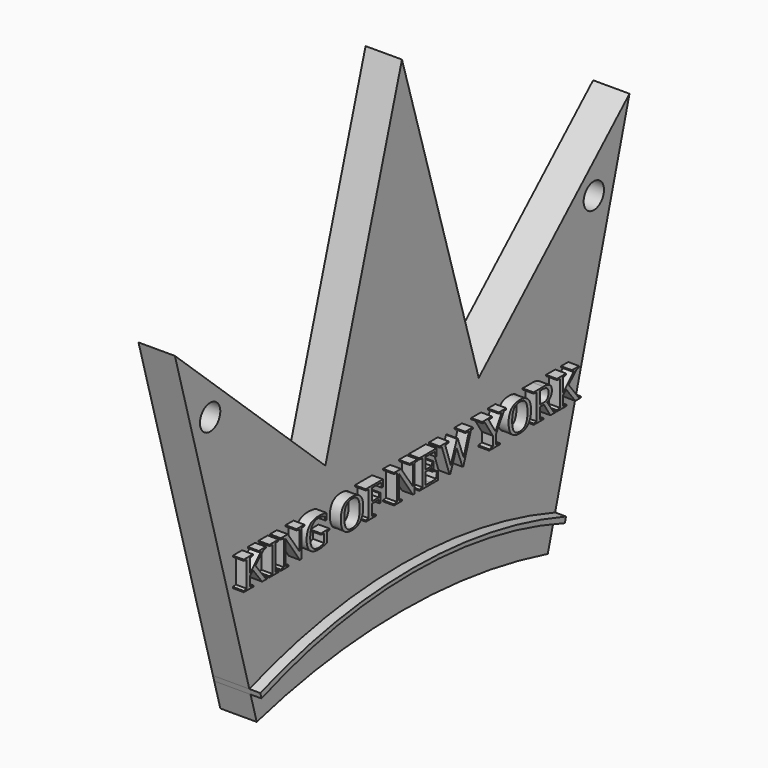
from build123d import *

# Parameters (mm, degrees)
F0_R         = 0.889
F1_DEPTH     = 2.54
F0_TEXT_SIZE = 3.0652309457
F2_DEPTH     = 3.302


# Not quite as in the source:
# - a feature names something its author has since deleted; it is built from what else it names
# - Text() gives the source's letters only with a copy of the font that has no kerning and outlines rounded to 1/6400 em; it was checked with that copy


with BuildPart() as f1:
    # F0 (on Right) → F1 (new body)
    with BuildSketch(Plane.YZ):
        with BuildLine():
            Line((-58.5731928543, 116.2585045769), (-59.2243112864, 116.8579392082))
            Line((-59.2243112864, 116.8579392082), (-52.7272009337, 93.7439392082))
            ThreePointArc((-52.7272009337, 93.7439392082), (-39.3847965103, 96.0063092306), (-26.0423920869, 93.7439392082))
            Line((-26.0423920869, 93.7439392082), (-19.5532767107, 116.8414972067))
            Line((-19.5532767107, 116.8414972067), (-32.7116451349, 104.7276000479))
            Line((-32.7116451349, 104.7276000479), (-39.408698678, 127.0142197609))
            Line((-39.408698678, 127.0142197609), (-46.0932555591, 104.7691867476))
            Line((-46.0932555591, 104.7691867476), (-58.5731928543, 116.2585045769))
        make_face()
        Polygon((-52.8586438159, 102.5280816539), (-52.230271472, 102.5280816539), (-52.230271472, 102.4485772262), (-52.4620795622, 102.4097828971), (-53.147446044, 101.7392636277), (-52.2901392639, 100.6405699106), (-52.073178386, 100.6003387544), (-52.073178386, 100.5208343267), (-52.5640942797, 100.5208343267), (-53.3495597095, 101.5357131352), (-53.6206410713, 101.3187522573), (-53.6206410713, 100.6405699106), (-53.3332756701, 100.6003387544), (-53.3332756701, 100.5208343267), (-54.1671142758, 100.5208343267), (-54.1671142758, 100.6003387544), (-53.9094432994, 100.6405699106), (-53.9094432994, 102.4097828971), (-54.1671142758, 102.4485772262), (-54.1671142758, 102.5280816539), (-53.3629700949, 102.5280816539), (-53.3629700949, 102.4485772262), (-53.6206410713, 102.4097828971), (-53.6206410713, 101.4638717849), (-52.6598827467, 102.4097828971), (-52.8586438159, 102.4485772262), align=None, mode=Mode.SUBTRACT)
        Polygon((-51.3858961349, 102.4097828971), (-51.3858961349, 100.6405699106), (-51.1287041008, 100.6003387544), (-51.1287041008, 100.5208343267), (-51.9309325124, 100.5208343267), (-51.9309325124, 100.6003387544), (-51.6732615361, 100.6405699106), (-51.6732615361, 102.4097828971), (-51.9309325124, 102.4485772262), (-51.9309325124, 102.5280816539), (-51.1287041008, 102.5280816539), (-51.1287041008, 102.4485772262), align=None, mode=Mode.SUBTRACT)
        Polygon((-49.2924391874, 101.0419235875), (-49.2924391874, 102.4097828971), (-49.5616047798, 102.4485772262), (-49.5616047798, 102.5280816539), (-48.8776751251, 102.5280816539), (-48.8776751251, 102.4485772262), (-49.1348671591, 102.4097828971), (-49.1348671591, 100.5208343267), (-49.280465629, 100.5208343267), (-50.5180526234, 102.3259679884), (-50.5180526234, 100.6405699106), (-50.2484080886, 100.6003387544), (-50.2484080886, 100.5208343267), (-50.9328166857, 100.5208343267), (-50.9328166857, 100.6003387544), (-50.6751457093, 100.6405699106), (-50.6751457093, 102.4097828971), (-50.9328166857, 102.4485772262), (-50.9328166857, 102.5280816539), (-50.3250388623, 102.5280816539), align=None, mode=Mode.SUBTRACT)
        with BuildLine():
            Line((-46.8852750103, 101.2780421588), (-46.8852750103, 100.6257226982))
            add(Edge.make_bspline(
                [(-46.8852750103, 100.6257226982), (-47.059131078, 100.5687285603), (-47.24615806, 100.5296947599)],
                knots=[0, 0, 0, 1, 1, 1], degree=2))
            add(Edge.make_bspline(
                [(-47.24615806, 100.5296947599), (-47.4331850419, 100.4906609596), (-47.6487090928, 100.4906609596)],
                knots=[0, 0, 0, 1, 1, 1], degree=2))
            add(Edge.make_bspline(
                [(-47.6487090928, 100.4906609596), (-48.1367513324, 100.4906609596), (-48.40903005, 100.7543187152)],
                knots=[0, 0, 0, 1, 1, 1], degree=2))
            add(Edge.make_bspline(
                [(-48.40903005, 100.7543187152), (-48.6813087676, 101.0179764708), (-48.6813087676, 101.501229287)],
                knots=[0, 0, 0, 1, 1, 1], degree=2))
            add(Edge.make_bspline(
                [(-48.6813087676, 101.501229287), (-48.6813087676, 102.0280658558), (-48.4171720697, 102.2893288997)],
                knots=[0, 0, 0, 1, 1, 1], degree=2))
            add(Edge.make_bspline(
                [(-48.4171720697, 102.2893288997), (-48.1530353718, 102.5505919436), (-47.6429617847, 102.5505919436)],
                knots=[0, 0, 0, 1, 1, 1], degree=2))
            add(Edge.make_bspline(
                [(-47.6429617847, 102.5505919436), (-47.2775287829, 102.5505919436), (-46.9379586672, 102.4605507846)],
                knots=[0, 0, 0, 1, 1, 1], degree=2))
            Line((-46.9379586672, 102.4605507846), (-46.9379586672, 102.0295026829))
            Line((-46.9379586672, 102.0295026829), (-47.0380576153, 102.0295026829))
            Line((-47.0380576153, 102.0295026829), (-47.0787677138, 102.2780737549))
            add(Edge.make_bspline(
                [(-47.0787677138, 102.2780737549), (-47.1817403159, 102.3513519322), (-47.3261414299, 102.391104146)],
                knots=[0, 0, 0, 1, 1, 1], degree=2))
            add(Edge.make_bspline(
                [(-47.3261414299, 102.391104146), (-47.470542544, 102.4308563598), (-47.6309882263, 102.4308563598)],
                knots=[0, 0, 0, 1, 1, 1], degree=2))
            add(Edge.make_bspline(
                [(-47.6309882263, 102.4308563598), (-48.0141420946, 102.4308563598), (-48.1913507586, 102.2024008659)],
                knots=[0, 0, 0, 1, 1, 1], degree=2))
            add(Edge.make_bspline(
                [(-48.1913507586, 102.2024008659), (-48.3685594227, 101.973945372), (-48.3685594227, 101.5041029411)],
                knots=[0, 0, 0, 1, 1, 1], degree=2))
            add(Edge.make_bspline(
                [(-48.3685594227, 101.5041029411), (-48.3685594227, 101.0625181079), (-48.1860823929, 100.8343020852)],
                knots=[0, 0, 0, 1, 1, 1], degree=2))
            add(Edge.make_bspline(
                [(-48.1860823929, 100.8343020852), (-48.0036053632, 100.6060860624), (-47.6458354387, 100.6060860624)],
                knots=[0, 0, 0, 1, 1, 1], degree=2))
            add(Edge.make_bspline(
                [(-47.6458354387, 100.6060860624), (-47.5198736046, 100.6060860624), (-47.3821776832, 100.6360199584)],
                knots=[0, 0, 0, 1, 1, 1], degree=2))
            add(Edge.make_bspline(
                [(-47.3821776832, 100.6360199584), (-47.2444817618, 100.6659538543), (-47.1726404115, 100.7081007798)],
                knots=[0, 0, 0, 1, 1, 1], degree=2))
            Line((-47.1726404115, 100.7081007798), (-47.1726404115, 101.2780421588))
            Line((-47.1726404115, 101.2780421588), (-47.4303113879, 101.3173154303))
            Line((-47.4303113879, 101.3173154303), (-47.4303113879, 101.3977777426))
            Line((-47.4303113879, 101.3977777426), (-46.6893875952, 101.3977777426))
            Line((-46.6893875952, 101.3977777426), (-46.6893875952, 101.3173154303))
            Line((-46.6893875952, 101.3173154303), (-46.8852750103, 101.2780421588))
        make_face(mode=Mode.SUBTRACT)
        with BuildLine():
            add(Edge.make_bspline(
                [(-45.4498848315, 100.7519240035), (-45.7013295575, 101.0131870474), (-45.7013295575, 101.5266132308)],
                knots=[0, 0, 0, 1, 1, 1], degree=2))
            add(Edge.make_bspline(
                [(-45.7013295575, 101.5266132308), (-45.7013295575, 102.5505919436), (-44.7214135396, 102.5505919436)],
                knots=[0, 0, 0, 1, 1, 1], degree=2))
            add(Edge.make_bspline(
                [(-44.7214135396, 102.5505919436), (-44.2362449539, 102.5505919436), (-43.9879133531, 102.2907657267)],
                knots=[0, 0, 0, 1, 1, 1], degree=2))
            add(Edge.make_bspline(
                [(-43.9879133531, 102.2907657267), (-43.7395817523, 102.0309395099), (-43.7395817523, 101.5266132308)],
                knots=[0, 0, 0, 1, 1, 1], degree=2))
            add(Edge.make_bspline(
                [(-43.7395817523, 101.5266132308), (-43.7395817523, 101.0146238744), (-43.9910264783, 100.752642417)],
                knots=[0, 0, 0, 1, 1, 1], degree=2))
            add(Edge.make_bspline(
                [(-43.9910264783, 100.752642417), (-44.2424712043, 100.4906609596), (-44.7214135396, 100.4906609596)],
                knots=[0, 0, 0, 1, 1, 1], degree=2))
            add(Edge.make_bspline(
                [(-44.7214135396, 100.4906609596), (-45.1984401055, 100.4906609596), (-45.4498848315, 100.7519240035)],
                knots=[0, 0, 0, 1, 1, 1], degree=2))
        make_face(mode=Mode.SUBTRACT)
        with BuildLine():
            Line((-42.3880064821, 101.4217248594), (-42.9790213238, 101.4217248594))
            Line((-42.9790213238, 101.4217248594), (-42.9790213238, 100.6405699106))
            Line((-42.9790213238, 100.6405699106), (-42.6451985162, 100.6003387544))
            Line((-42.6451985162, 100.6003387544), (-42.6451985162, 100.5208343267))
            Line((-42.6451985162, 100.5208343267), (-43.5058578926, 100.5208343267))
            Line((-43.5058578926, 100.5208343267), (-43.5058578926, 100.6003387544))
            Line((-43.5058578926, 100.6003387544), (-43.267823552, 100.6405699106))
            Line((-43.267823552, 100.6405699106), (-43.267823552, 102.4097828971))
            Line((-43.267823552, 102.4097828971), (-43.5254945284, 102.4485772262))
            Line((-43.5254945284, 102.4485772262), (-43.5254945284, 102.5280816539))
            Line((-43.5254945284, 102.5280816539), (-42.0196998263, 102.5280816539))
            Line((-42.0196998263, 102.5280816539), (-42.0196998263, 102.0477024916))
            Line((-42.0196998263, 102.0477024916), (-42.1183619474, 102.0477024916))
            Line((-42.1183619474, 102.0477024916), (-42.1662561809, 102.3724253949))
            add(Edge.make_bspline(
                [(-42.1662561809, 102.3724253949), (-42.3338859982, 102.3930199153), (-42.6514247665, 102.3930199153)],
                knots=[0, 0, 0, 1, 1, 1], degree=2))
            Line((-42.6514247665, 102.3930199153), (-42.9790213238, 102.3930199153))
            Line((-42.9790213238, 102.3930199153), (-42.9790213238, 101.5567865979))
            Line((-42.9790213238, 101.5567865979), (-42.3880064821, 101.5567865979))
            Line((-42.3880064821, 101.5567865979), (-42.3415490756, 101.7962577656))
            Line((-42.3415490756, 101.7962577656), (-42.2500710896, 101.7962577656))
            Line((-42.2500710896, 101.7962577656), (-42.2500710896, 101.1793800377))
            Line((-42.2500710896, 101.1793800377), (-42.3415490756, 101.1793800377))
            Line((-42.3415490756, 101.1793800377), (-42.3880064821, 101.4217248594))
        make_face(mode=Mode.SUBTRACT)
        Polygon((-39.4142535224, 101.0419235875), (-39.4142535224, 102.4097828971), (-39.6834191148, 102.4485772262), (-39.6834191148, 102.5280816539), (-38.9994894601, 102.5280816539), (-38.9994894601, 102.4485772262), (-39.2566814941, 102.4097828971), (-39.2566814941, 100.5208343267), (-39.402279964, 100.5208343267), (-40.6398669584, 102.3259679884), (-40.6398669584, 100.6405699106), (-40.3702224236, 100.6003387544), (-40.3702224236, 100.5208343267), (-41.0546310207, 100.5208343267), (-41.0546310207, 100.6003387544), (-40.7969600443, 100.6405699106), (-40.7969600443, 102.4097828971), (-41.0546310207, 102.4485772262), (-41.0546310207, 102.5280816539), (-40.4468531973, 102.5280816539), align=None, mode=Mode.SUBTRACT)
        with BuildLine():
            Line((-38.8409595471, 100.5208343267), (-38.8409595471, 100.6003387544))
            Line((-38.8409595471, 100.6003387544), (-38.5832885707, 100.6405699106))
            Line((-38.5832885707, 100.6405699106), (-38.5832885707, 102.4097828971))
            Line((-38.5832885707, 102.4097828971), (-38.8409595471, 102.4485772262))
            Line((-38.8409595471, 102.4485772262), (-38.8409595471, 102.5280816539))
            Line((-38.8409595471, 102.5280816539), (-37.335164845, 102.5280816539))
            Line((-37.335164845, 102.5280816539), (-37.335164845, 102.0477024916))
            Line((-37.335164845, 102.0477024916), (-37.4338269661, 102.0477024916))
            Line((-37.4338269661, 102.0477024916), (-37.4817211996, 102.3724253949))
            add(Edge.make_bspline(
                [(-37.4817211996, 102.3724253949), (-37.6493510169, 102.3930199153), (-37.9668897852, 102.3930199153)],
                knots=[0, 0, 0, 1, 1, 1], degree=2))
            Line((-37.9668897852, 102.3930199153), (-38.2944863425, 102.3930199153))
            Line((-38.2944863425, 102.3930199153), (-38.2944863425, 101.6089913125))
            Line((-38.2944863425, 101.6089913125), (-37.7528025613, 101.6089913125))
            Line((-37.7528025613, 101.6089913125), (-37.7063451548, 101.8484624801))
            Line((-37.7063451548, 101.8484624801), (-37.6105566878, 101.8484624801))
            Line((-37.6105566878, 101.8484624801), (-37.6105566878, 101.2315847523))
            Line((-37.6105566878, 101.2315847523), (-37.7063451548, 101.2315847523))
            Line((-37.7063451548, 101.2315847523), (-37.7528025613, 101.4744085163))
            Line((-37.7528025613, 101.4744085163), (-38.2944863425, 101.4744085163))
            Line((-38.2944863425, 101.4744085163), (-38.2944863425, 100.655417123))
            Line((-38.2944863425, 100.655417123), (-37.8993589159, 100.655417123))
            add(Edge.make_bspline(
                [(-37.8993589159, 100.655417123), (-37.5133313937, 100.655417123), (-37.3935958099, 100.6793642397)],
                knots=[0, 0, 0, 1, 1, 1], degree=2))
            Line((-37.3935958099, 100.6793642397), (-37.3083440742, 101.0505445496))
            Line((-37.3083440742, 101.0505445496), (-37.2092030108, 101.0505445496))
            Line((-37.2092030108, 101.0505445496), (-37.2379395509, 100.5208343267))
            Line((-37.2379395509, 100.5208343267), (-38.8409595471, 100.5208343267))
        make_face(mode=Mode.SUBTRACT)
        Polygon((-34.3446489035, 102.4097828971), (-35.0003209605, 100.4743769202), (-35.0798253882, 100.4743769202), (-35.6004357066, 101.8575623845), (-36.1349353528, 100.4743769202), (-36.2144397805, 100.4743769202), (-36.8787327995, 102.4097828971), (-37.0540256942, 102.4485772262), (-37.0540256942, 102.5280816539), (-36.2877179577, 102.5280816539), (-36.2877179577, 102.4485772262), (-36.5822674939, 102.4097828971), (-36.1047619857, 100.995466181), (-35.5645150315, 102.3872726073), (-35.4974631045, 102.3872726073), (-34.9763738438, 100.995466181), (-34.5213786253, 102.4097828971), (-34.8341279702, 102.4485772262), (-34.8341279702, 102.5280816539), (-34.1698349512, 102.5280816539), (-34.1698349512, 102.4485772262), align=None, mode=Mode.SUBTRACT)
        Polygon((-31.4815316233, 102.4097828971), (-32.1429509883, 101.3110891799), (-32.1429509883, 100.6405699106), (-31.8244543353, 100.6003387544), (-31.8244543353, 100.5208343267), (-32.7507288118, 100.5208343267), (-32.7507288118, 100.6003387544), (-32.4317532165, 100.6405699106), (-32.4317532165, 101.3019892756), (-33.136756334, 102.4097828971), (-33.3628171162, 102.4485772262), (-33.3628171162, 102.5280816539), (-32.5141312981, 102.5280816539), (-32.5141312981, 102.4485772262), (-32.7837758329, 102.4097828971), (-32.2076082036, 101.4830294783), (-31.659698172, 102.4097828971), (-31.914016552, 102.4485772262), (-31.914016552, 102.5280816539), (-31.2616970914, 102.5280816539), (-31.2616970914, 102.4485772262), align=None, mode=Mode.SUBTRACT)
        with BuildLine():
            add(Edge.make_bspline(
                [(-30.8062229306, 100.7519240035), (-31.0576676566, 101.0131870474), (-31.0576676566, 101.5266132308)],
                knots=[0, 0, 0, 1, 1, 1], degree=2))
            add(Edge.make_bspline(
                [(-31.0576676566, 101.5266132308), (-31.0576676566, 102.5505919436), (-30.0777516386, 102.5505919436)],
                knots=[0, 0, 0, 1, 1, 1], degree=2))
            add(Edge.make_bspline(
                [(-30.0777516386, 102.5505919436), (-29.592583053, 102.5505919436), (-29.3442514521, 102.2907657267)],
                knots=[0, 0, 0, 1, 1, 1], degree=2))
            add(Edge.make_bspline(
                [(-29.3442514521, 102.2907657267), (-29.0959198513, 102.0309395099), (-29.0959198513, 101.5266132308)],
                knots=[0, 0, 0, 1, 1, 1], degree=2))
            add(Edge.make_bspline(
                [(-29.0959198513, 101.5266132308), (-29.0959198513, 101.0146238744), (-29.3473645773, 100.752642417)],
                knots=[0, 0, 0, 1, 1, 1], degree=2))
            add(Edge.make_bspline(
                [(-29.3473645773, 100.752642417), (-29.5988093033, 100.4906609596), (-30.0777516386, 100.4906609596)],
                knots=[0, 0, 0, 1, 1, 1], degree=2))
            add(Edge.make_bspline(
                [(-30.0777516386, 100.4906609596), (-30.5547782045, 100.4906609596), (-30.8062229306, 100.7519240035)],
                knots=[0, 0, 0, 1, 1, 1], degree=2))
        make_face(mode=Mode.SUBTRACT)
        with BuildLine():
            Line((-27.9747158444, 101.401130339), (-28.3353594229, 101.401130339))
            Line((-28.3353594229, 101.401130339), (-28.3353594229, 100.6405699106))
            Line((-28.3353594229, 100.6405699106), (-28.0317099823, 100.6003387544))
            Line((-28.0317099823, 100.6003387544), (-28.0317099823, 100.5208343267))
            Line((-28.0317099823, 100.5208343267), (-28.8621959917, 100.5208343267))
            Line((-28.8621959917, 100.5208343267), (-28.8621959917, 100.6003387544))
            Line((-28.8621959917, 100.6003387544), (-28.624161651, 100.6405699106))
            Line((-28.624161651, 100.6405699106), (-28.624161651, 102.4097828971))
            Line((-28.624161651, 102.4097828971), (-28.8818326274, 102.4485772262))
            Line((-28.8818326274, 102.4485772262), (-28.8818326274, 102.5280816539))
            Line((-28.8818326274, 102.5280816539), (-28.0149470006, 102.5280816539))
            add(Edge.make_bspline(
                [(-28.0149470006, 102.5280816539), (-27.6380193827, 102.5280816539), (-27.458416007, 102.4006829927)],
                knots=[0, 0, 0, 1, 1, 1], degree=2))
            add(Edge.make_bspline(
                [(-27.458416007, 102.4006829927), (-27.2788126313, 102.2732843315), (-27.2788126313, 101.9921451807)],
                knots=[0, 0, 0, 1, 1, 1], degree=2))
            add(Edge.make_bspline(
                [(-27.2788126313, 101.9921451807), (-27.2788126313, 101.7914683422), (-27.3880114837, 101.6456304011)],
                knots=[0, 0, 0, 1, 1, 1], degree=2))
            add(Edge.make_bspline(
                [(-27.3880114837, 101.6456304011), (-27.4972103362, 101.49979246), (-27.6902240973, 101.4427983221)],
                knots=[0, 0, 0, 1, 1, 1], degree=2))
            Line((-27.6902240973, 101.4427983221), (-27.1471034891, 100.6405699106))
            Line((-27.1471034891, 100.6405699106), (-26.9301426112, 100.6003387544))
            Line((-26.9301426112, 100.6003387544), (-26.9301426112, 100.5208343267))
            Line((-26.9301426112, 100.5208343267), (-27.4105217735, 100.5208343267))
            Line((-27.4105217735, 100.5208343267), (-27.9747158444, 101.401130339))
        make_face(mode=Mode.SUBTRACT)
        Polygon((-25.5287573382, 102.5280816539), (-24.9003849943, 102.5280816539), (-24.9003849943, 102.4485772262), (-25.1321930846, 102.4097828971), (-25.8175595663, 101.7392636277), (-24.9602527862, 100.6405699106), (-24.7432919083, 100.6003387544), (-24.7432919083, 100.5208343267), (-25.234207802, 100.5208343267), (-26.0196732318, 101.5357131352), (-26.2907545936, 101.3187522573), (-26.2907545936, 100.6405699106), (-26.0033891924, 100.6003387544), (-26.0033891924, 100.5208343267), (-26.8372277981, 100.5208343267), (-26.8372277981, 100.6003387544), (-26.5795568218, 100.6405699106), (-26.5795568218, 102.4097828971), (-26.8372277981, 102.4485772262), (-26.8372277981, 102.5280816539), (-26.0330836172, 102.5280816539), (-26.0330836172, 102.4485772262), (-26.2907545936, 102.4097828971), (-26.2907545936, 101.4638717849), (-25.329996269, 102.4097828971), (-25.5287573382, 102.4485772262), align=None, mode=Mode.SUBTRACT)
        with Locations((-56.149866432, 111.8401065469)):
            Circle(F0_R, mode=Mode.SUBTRACT)
        with Locations((-22.6675309241, 111.8401065469)):
            Circle(F0_R, mode=Mode.SUBTRACT)
        with BuildLine():
            ThreePointArc((-26.0423920869, 93.7439392082), (-39.3847965103, 96.0063092306), (-52.7272009337, 93.7439392082))
            Line((-52.7272009337, 93.7439392082), (-52.6201057081, 93.3629392082))
            ThreePointArc((-52.6201057081, 93.3629392082), (-39.384040312, 95.7310608711), (-26.1454420616, 93.3771399406))
            Line((-26.1454420616, 93.3771399406), (-26.0423920869, 93.7439392082))
        make_face()
        with BuildLine():
            ThreePointArc((-26.1454420616, 93.3771399406), (-39.384040312, 95.7310608711), (-52.6201057081, 93.3629392082))
            Line((-52.6201057081, 93.3629392082), (-52.0846295802, 91.4579392082))
            ThreePointArc((-52.0846295802, 91.4579392082), (-39.3846295802, 93.1373896631), (-26.6846295802, 91.4579392082))
            Line((-26.6846295802, 91.4579392082), (-26.1454420616, 93.3771399406))
        make_face()
    extrude(amount=F1_DEPTH)


with BuildPart() as f1b:
    # F0 (on Right) → F1, piece 2 (new body)
    with BuildSketch(Plane.YZ):
        with BuildLine():
            add(Edge.make_bspline(
                [(-45.227655588, 102.2189243765), (-45.3885802126, 102.0069923931), (-45.3885802126, 101.5266132308)],
                knots=[0, 0, 0, 1, 1, 1], degree=2))
            add(Edge.make_bspline(
                [(-45.3885802126, 101.5266132308), (-45.3885802126, 101.0433604145), (-45.2269371744, 100.8261600655)],
                knots=[0, 0, 0, 1, 1, 1], degree=2))
            add(Edge.make_bspline(
                [(-45.2269371744, 100.8261600655), (-45.0652941363, 100.6089597164), (-44.7214135396, 100.6089597164)],
                knots=[0, 0, 0, 1, 1, 1], degree=2))
            add(Edge.make_bspline(
                [(-44.7214135396, 100.6089597164), (-44.3784908275, 100.6089597164), (-44.2154109624, 100.8261600655)],
                knots=[0, 0, 0, 1, 1, 1], degree=2))
            add(Edge.make_bspline(
                [(-44.2154109624, 100.8261600655), (-44.0523310972, 101.0433604145), (-44.0523310972, 101.5266132308)],
                knots=[0, 0, 0, 1, 1, 1], degree=2))
            add(Edge.make_bspline(
                [(-44.0523310972, 101.5266132308), (-44.0523310972, 102.0069923931), (-44.2146925488, 102.2189243765)],
                knots=[0, 0, 0, 1, 1, 1], degree=2))
            add(Edge.make_bspline(
                [(-44.2146925488, 102.2189243765), (-44.3770540005, 102.4308563598), (-44.7214135396, 102.4308563598)],
                knots=[0, 0, 0, 1, 1, 1], degree=2))
            add(Edge.make_bspline(
                [(-44.7214135396, 102.4308563598), (-45.0667309633, 102.4308563598), (-45.227655588, 102.2189243765)],
                knots=[0, 0, 0, 1, 1, 1], degree=2))
        make_face()
    extrude(amount=F1_DEPTH)


with BuildPart() as f1c:
    # F0 (on Right) → F1, piece 3 (new body)
    with BuildSketch(Plane.YZ):
        with BuildLine():
            add(Edge.make_bspline(
                [(-30.583993687, 102.2189243765), (-30.7449183116, 102.0069923931), (-30.7449183116, 101.5266132308)],
                knots=[0, 0, 0, 1, 1, 1], degree=2))
            add(Edge.make_bspline(
                [(-30.7449183116, 101.5266132308), (-30.7449183116, 101.0433604145), (-30.5832752735, 100.8261600655)],
                knots=[0, 0, 0, 1, 1, 1], degree=2))
            add(Edge.make_bspline(
                [(-30.5832752735, 100.8261600655), (-30.4216322353, 100.6089597164), (-30.0777516386, 100.6089597164)],
                knots=[0, 0, 0, 1, 1, 1], degree=2))
            add(Edge.make_bspline(
                [(-30.0777516386, 100.6089597164), (-29.7348289265, 100.6089597164), (-29.5717490614, 100.8261600655)],
                knots=[0, 0, 0, 1, 1, 1], degree=2))
            add(Edge.make_bspline(
                [(-29.5717490614, 100.8261600655), (-29.4086691962, 101.0433604145), (-29.4086691962, 101.5266132308)],
                knots=[0, 0, 0, 1, 1, 1], degree=2))
            add(Edge.make_bspline(
                [(-29.4086691962, 101.5266132308), (-29.4086691962, 102.0069923931), (-29.5710306479, 102.2189243765)],
                knots=[0, 0, 0, 1, 1, 1], degree=2))
            add(Edge.make_bspline(
                [(-29.5710306479, 102.2189243765), (-29.7333920995, 102.4308563598), (-30.0777516386, 102.4308563598)],
                knots=[0, 0, 0, 1, 1, 1], degree=2))
            add(Edge.make_bspline(
                [(-30.0777516386, 102.4308563598), (-30.4230690623, 102.4308563598), (-30.583993687, 102.2189243765)],
                knots=[0, 0, 0, 1, 1, 1], degree=2))
        make_face()
    extrude(amount=F1_DEPTH)


with BuildPart() as f1d:
    # F0 (on Right) → F1, piece 4 (new body)
    with BuildSketch(Plane.YZ):
        with BuildLine():
            add(Edge.make_bspline(
                [(-27.6895056838, 101.6350936698), (-27.5767147638, 101.7344742043), (-27.5767147638, 101.971071718)],
                knots=[0, 0, 0, 1, 1, 1], degree=2))
            add(Edge.make_bspline(
                [(-27.5767147638, 101.971071718), (-27.5767147638, 102.2000061542), (-27.6880688568, 102.2965130348)],
                knots=[0, 0, 0, 1, 1, 1], degree=2))
            add(Edge.make_bspline(
                [(-27.6880688568, 102.2965130348), (-27.7994229497, 102.3930199153), (-28.0796042158, 102.3930199153)],
                knots=[0, 0, 0, 1, 1, 1], degree=2))
            Line((-28.0796042158, 102.3930199153), (-28.3353594229, 102.3930199153))
            Line((-28.3353594229, 102.3930199153), (-28.3353594229, 101.5357131352))
            Line((-28.3353594229, 101.5357131352), (-28.0705043115, 101.5357131352))
            add(Edge.make_bspline(
                [(-28.0705043115, 101.5357131352), (-27.8022966037, 101.5357131352), (-27.6895056838, 101.6350936698)],
                knots=[0, 0, 0, 1, 1, 1], degree=2))
        make_face()
    extrude(amount=F1_DEPTH)


with BuildPart() as f2:
    # F0 (on Right) → F2 (new body)
    with BuildSketch(Plane.YZ):
        with Locations((-54.2552396655, 100.5208343267)):
            Text('KING OF NEW YORK', F0_TEXT_SIZE, font='Tinos', text_align=(TextAlign.LEFT, TextAlign.BOTTOM))
        with BuildLine():
            ThreePointArc((-26.0423920869, 93.7439392082), (-39.3847965103, 96.0063092306), (-52.7272009337, 93.7439392082))
            Line((-52.7272009337, 93.7439392082), (-52.6201057081, 93.3629392082))
            ThreePointArc((-52.6201057081, 93.3629392082), (-39.384040312, 95.7310608711), (-26.1454420616, 93.3771399406))
            Line((-26.1454420616, 93.3771399406), (-26.0423920869, 93.7439392082))
        make_face()
    extrude(amount=F2_DEPTH)


solid = Compound([f1.part, f1b.part, f1c.part, f1d.part, f2.part])
